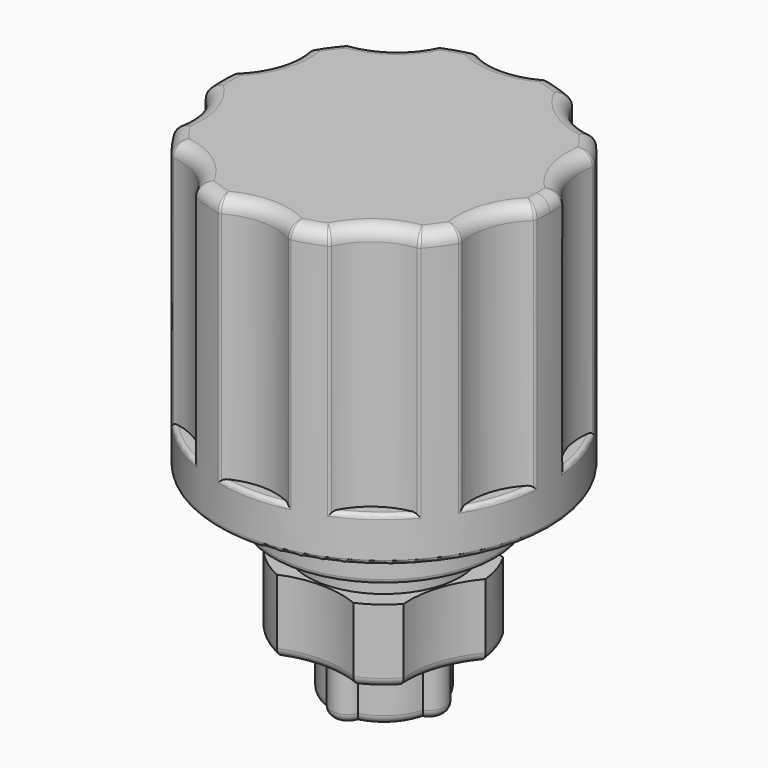
from build123d import *

# Parameters (mm, degrees)
F0_R         = 9.398
F1_DEPTH     = 16.51
F2_R         = 3.81
F3_DEPTH     = 13.97
F4_T2_ANGLE  = 17.4807543579
F4_T4_ANGLE  = 17.4807543579
F4_T6_ANGLE  = 119.7648433204
F4_T8_ANGLE  = 34.9616276293
F4_T10_ANGLE = 119.7648433204
F4_T12_ANGLE = 34.9616276293
F4_T14_ANGLE = 119.7648433204
F4_T16_ANGLE = 34.9616276293
F4_T18_ANGLE = 119.7648433204
F4_T20_ANGLE = 34.9616276293
F4_T22_ANGLE = 119.7648433204
F4_T24_ANGLE = 34.9616276293
F4_T26_ANGLE = 119.7648433204
F4_T28_ANGLE = 34.9616276293
F4_T30_ANGLE = 119.7648433204
F4_T32_ANGLE = 34.9616276293
F4_T34_ANGLE = 119.7648433204
F4_T36_ANGLE = 34.9616276293
F4_T38_ANGLE = 119.7648433204
F4_T40_ANGLE = 34.9616276293
F4_T42_ANGLE = 119.7648433204
F5_R         = 5.334
F6_DEPTH     = 8.255
F7_R         = 5.715
F8_DEPTH     = 7.62
F9_R         = 6.223
F9_R_2       = 4.3172960793
F10_DEPTH    = 4.064
F11_R        = 6.35
F12_DEPTH    = 2.54
F13_R        = 0.508
F14_R        = 0.254
F15_R        = 1.524
F16_DEPTH    = 10.414
F17_R        = 1.524
F18_DEPTH    = 3.048
F19_R        = 0.508


# Not quite as in the source:
# - a fillet or chamfer that OpenCascade refuses, or shapes differently, is made with other operations: its cross-section is extruded or revolved along the edge and cut away or added


with BuildPart() as f1:
    # F0 (on Top) → F1 (new body)
    with BuildSketch(Plane.XY):
        Circle(F0_R)
    extrude(amount=F1_DEPTH)

    # F2 (on face) → F3 (cut)
    with BuildSketch(Plane.XY.offset(16.51)):
        with Locations((-7.31557525, 10.069025512)):
            Circle(F2_R)
        with Locations((-11.8368494018, 3.846025512)):
            Circle(F2_R)
        with Locations((-11.8368494018, -3.846025512)):
            Circle(F2_R)
        with Locations((-7.31557525, -10.069025512)):
            Circle(F2_R)
        with Locations((0, -12.446)):
            Circle(F2_R)
        with Locations((7.31557525, -10.069025512)):
            Circle(F2_R)
        with Locations((11.8368494018, -3.846025512)):
            Circle(F2_R)
        with Locations((11.8368494018, 3.846025512)):
            Circle(F2_R)
        with Locations((7.31557525, 10.069025512)):
            Circle(F2_R)
        with Locations((0, 12.446)):
            Circle(F2_R)
    extrude(amount=-F3_DEPTH, mode=Mode.SUBTRACT)

    # F4: fillet of radius 0.762 on 21 edges, made by hand

    # F4_s1 → F4_t2 (revolve, cut)
    with BuildSketch(Plane(origin=(0, 0, 0), x_dir=(0, 0, 1), z_dir=(-0.3003854292, -0.953817904, 0))):
        with BuildLine():
            ThreePointArc((15.748, -9.398), (16.2868153673, -9.1748153673), (16.51, -8.636))
            Line((16.51, -8.636), (16.51, -9.398))
            Line((16.51, -9.398), (15.748, -9.398))
        make_face()
    revolve(axis=Axis((0, 0, 16.51), (0, 0, 1)), revolution_arc=F4_T2_ANGLE, mode=Mode.SUBTRACT)

    # F4_s3 → F4_t4 (revolve, cut)
    with BuildSketch(Plane.XZ):
        with BuildLine():
            ThreePointArc((9.398, 15.748), (9.1748153673, 16.2868153673), (8.636, 16.51))
            Line((8.636, 16.51), (9.398, 16.51))
            Line((9.398, 16.51), (9.398, 15.748))
        make_face()
    revolve(axis=Axis((0, 0, 16.51), (0, 0, 1)), revolution_arc=F4_T4_ANGLE, mode=Mode.SUBTRACT)

    # F4_s5 → F4_t6 (revolve, cut)
    with BuildSketch(Plane(origin=(7.187265654, 8.0152842237, 0), x_dir=(0, 0, 1), z_dir=(0.6676041693, 0.7445164022, 0))):
        with BuildLine():
            ThreePointArc((15.748, 2.4351058624), (16.2868153673, 2.2119212297), (16.51, 1.6731058624))
            Line((16.51, 1.6731058624), (16.51, 2.4351058624))
            Line((16.51, 2.4351058624), (15.748, 2.4351058624))
        make_face()
    revolve(axis=Axis((11.8368494018, 3.846025512, 16.51), (0, 0, 1)), revolution_arc=F4_T6_ANGLE, mode=Mode.SUBTRACT)

    # F4_s7 → F4_t8 (revolve, cut)
    with BuildSketch(Plane(origin=(0, 0, 0), x_dir=(0, 0, 1), z_dir=(0.3176221963, -0.9482173487, 0))):
        with BuildLine():
            ThreePointArc((15.748, -9.398), (16.2868153673, -9.1748153673), (16.51, -8.636))
            Line((16.51, -8.636), (16.51, -9.398))
            Line((16.51, -9.398), (15.748, -9.398))
        make_face()
    revolve(axis=Axis((0, 0, 16.51), (0, 0, 1)), revolution_arc=F4_T8_ANGLE, mode=Mode.SUBTRACT)

    # F4_s9 → F4_t10 (revolve, cut)
    with BuildSketch(Plane(origin=(1.1033541976, 10.7090699074, 0), x_dir=(0, 0, 1), z_dir=(0.1024873572, 0.994734307, 0))):
        with BuildLine():
            ThreePointArc((15.748, 2.4351058624), (16.2868153673, 2.2119212297), (16.51, 1.6731058624))
            Line((16.51, 1.6731058624), (16.51, 2.4351058624))
            Line((16.51, 2.4351058624), (15.748, 2.4351058624))
        make_face()
    revolve(axis=Axis((7.31557525, 10.069025512, 16.51), (0, 0, 1)), revolution_arc=F4_T10_ANGLE, mode=Mode.SUBTRACT)

    # F4_s11 → F4_t12 (revolve, cut)
    with BuildSketch(Plane(origin=(0, 0, 0), x_dir=(0, 0, 1), z_dir=(0.8143099281, -0.5804303067, 0))):
        with BuildLine():
            ThreePointArc((15.748, -9.398), (16.2868153673, -9.1748153673), (16.51, -8.636))
            Line((16.51, -8.636), (16.51, -9.398))
            Line((16.51, -9.398), (15.748, -9.398))
        make_face()
    revolve(axis=Axis((0, 0, 16.51), (0, 0, 1)), revolution_arc=F4_T12_ANGLE, mode=Mode.SUBTRACT)

    # F4_s13 → F4_t14 (revolve, cut)
    with BuildSketch(Plane(origin=(-5.4020010607, 9.3123548744, 0), x_dir=(0, 0, 1), z_dir=(-0.5017761419, 0.8649975164, 0))):
        with BuildLine():
            ThreePointArc((15.748, 2.4351058624), (16.2868153673, 2.2119212297), (16.51, 1.6731058624))
            Line((16.51, 1.6731058624), (16.51, 2.4351058624))
            Line((16.51, 2.4351058624), (15.748, 2.4351058624))
        make_face()
    revolve(axis=Axis((0, 12.446, 16.51), (0, 0, 1)), revolution_arc=F4_T14_ANGLE, mode=Mode.SUBTRACT)

    # F4_s15 → F4_t16 (revolve, cut)
    with BuildSketch(Plane(origin=(0, 0, 0), x_dir=(0, 0, 1), z_dir=(0.9999589448, 0.0090613844, 0))):
        with BuildLine():
            ThreePointArc((15.748, -9.398), (16.2868153673, -9.1748153673), (16.51, -8.636))
            Line((16.51, -8.636), (16.51, -9.398))
            Line((16.51, -9.398), (15.748, -9.398))
        make_face()
    revolve(axis=Axis((0, 0, 16.51), (0, 0, 1)), revolution_arc=F4_T16_ANGLE, mode=Mode.SUBTRACT)

    # F4_s17 → F4_t18 (revolve, cut)
    with BuildSketch(Plane(origin=(-9.843975521, 4.3586367947, 0), x_dir=(0, 0, 1), z_dir=(-0.9143782096, 0.4048610747, 0))):
        with BuildLine():
            ThreePointArc((15.748, 2.4351058624), (16.2868153673, 2.2119212297), (16.51, 1.6731058624))
            Line((16.51, 1.6731058624), (16.51, 2.4351058624))
            Line((16.51, 2.4351058624), (15.748, 2.4351058624))
        make_face()
    revolve(axis=Axis((-7.31557525, 10.069025512, 16.51), (0, 0, 1)), revolution_arc=F4_T18_ANGLE, mode=Mode.SUBTRACT)

    # F4_s19 → F4_t20 (revolve, cut)
    with BuildSketch(Plane(origin=(0, 0, 0), x_dir=(0, 0, 1), z_dir=(0.8036576319, 0.5950919346, 0))):
        with BuildLine():
            ThreePointArc((15.748, -9.398), (16.2868153673, -9.1748153673), (16.51, -8.636))
            Line((16.51, -8.636), (16.51, -9.398))
            Line((16.51, -9.398), (15.748, -9.398))
        make_face()
    revolve(axis=Axis((0, 0, 16.51), (0, 0, 1)), revolution_arc=F4_T20_ANGLE, mode=Mode.SUBTRACT)

    # F4_s21 → F4_t22 (revolve, cut)
    with BuildSketch(Plane(origin=(-7.187265654, 8.0152842237, 0), x_dir=(0, 0, 1), z_dir=(-0.6676041693, 0.7445164022, 0))):
        with BuildLine():
            ThreePointArc((15.748, -2.4351058624), (16.2868153673, -2.2119212297), (16.51, -1.6731058624))
            Line((16.51, -1.6731058624), (16.51, -2.4351058624))
            Line((16.51, -2.4351058624), (15.748, -2.4351058624))
        make_face()
    revolve(axis=Axis((-11.8368494018, 3.846025512, 16.51), (0, 0, -1)), revolution_arc=F4_T22_ANGLE, mode=Mode.SUBTRACT)

    # F4_s23 → F4_t24 (revolve, cut)
    with BuildSketch(Plane(origin=(0, 0, 0), x_dir=(0, 0, 1), z_dir=(0.300386419, 0.9538175923, 0))):
        with BuildLine():
            ThreePointArc((15.748, -9.398), (16.2868153673, -9.1748153673), (16.51, -8.636))
            Line((16.51, -8.636), (16.51, -9.398))
            Line((16.51, -9.398), (15.748, -9.398))
        make_face()
    revolve(axis=Axis((0, 0, 16.51), (0, 0, 1)), revolution_arc=F4_T24_ANGLE, mode=Mode.SUBTRACT)

    # F4_s25 → F4_t26 (revolve, cut)
    with BuildSketch(Plane(origin=(-10.5258859168, 2.259932396, 0), x_dir=(0, 0, 1), z_dir=(-0.9777188798, 0.2099185368, 0))):
        with BuildLine():
            ThreePointArc((15.748, -2.4351058624), (16.2868153673, -2.2119212297), (16.51, -1.6731058624))
            Line((16.51, -1.6731058624), (16.51, -2.4351058624))
            Line((16.51, -2.4351058624), (15.748, -2.4351058624))
        make_face()
    revolve(axis=Axis((-11.8368494018, -3.846025512, 16.51), (0, 0, -1)), revolution_arc=F4_T26_ANGLE, mode=Mode.SUBTRACT)

    # F4_s27 → F4_t28 (revolve, cut)
    with BuildSketch(Plane(origin=(0, 0, 0), x_dir=(0, 0, 1), z_dir=(-0.3176221963, 0.9482173487, 0))):
        with BuildLine():
            ThreePointArc((15.748, -9.398), (16.2868153673, -9.1748153673), (16.51, -8.636))
            Line((16.51, -8.636), (16.51, -9.398))
            Line((16.51, -9.398), (15.748, -9.398))
        make_face()
    revolve(axis=Axis((0, 0, 16.51), (0, 0, 1)), revolution_arc=F4_T28_ANGLE, mode=Mode.SUBTRACT)

    # F4_s29 → F4_t30 (revolve, cut)
    with BuildSketch(Plane(origin=(-1.1033541976, -10.7090699074, 0), x_dir=(0, 0, 1), z_dir=(-0.1024873572, -0.994734307, 0))):
        with BuildLine():
            ThreePointArc((15.748, 2.4351058624), (16.2868153673, 2.2119212297), (16.51, 1.6731058624))
            Line((16.51, 1.6731058624), (16.51, 2.4351058624))
            Line((16.51, 2.4351058624), (15.748, 2.4351058624))
        make_face()
    revolve(axis=Axis((-7.31557525, -10.069025512, 16.51), (0, 0, 1)), revolution_arc=F4_T30_ANGLE, mode=Mode.SUBTRACT)

    # F4_s31 → F4_t32 (revolve, cut)
    with BuildSketch(Plane(origin=(0, 0, 0), x_dir=(0, 0, 1), z_dir=(-0.8143099281, 0.5804303067, 0))):
        with BuildLine():
            ThreePointArc((15.748, -9.398), (16.2868153673, -9.1748153673), (16.51, -8.636))
            Line((16.51, -8.636), (16.51, -9.398))
            Line((16.51, -9.398), (15.748, -9.398))
        make_face()
    revolve(axis=Axis((0, 0, 16.51), (0, 0, 1)), revolution_arc=F4_T32_ANGLE, mode=Mode.SUBTRACT)

    # F4_s33 → F4_t34 (revolve, cut)
    with BuildSketch(Plane(origin=(5.4020010607, -9.3123548744, 0), x_dir=(0, 0, 1), z_dir=(0.5017761419, -0.8649975164, 0))):
        with BuildLine():
            ThreePointArc((15.748, 2.4351058624), (16.2868153673, 2.2119212297), (16.51, 1.6731058624))
            Line((16.51, 1.6731058624), (16.51, 2.4351058624))
            Line((16.51, 2.4351058624), (15.748, 2.4351058624))
        make_face()
    revolve(axis=Axis((0, -12.446, 16.51), (0, 0, 1)), revolution_arc=F4_T34_ANGLE, mode=Mode.SUBTRACT)

    # F4_s35 → F4_t36 (revolve, cut)
    with BuildSketch(Plane(origin=(0, 0, 0), x_dir=(0, 0, 1), z_dir=(-0.9999589448, -0.0090613844, 0))):
        with BuildLine():
            ThreePointArc((15.748, -9.398), (16.2868153673, -9.1748153673), (16.51, -8.636))
            Line((16.51, -8.636), (16.51, -9.398))
            Line((16.51, -9.398), (15.748, -9.398))
        make_face()
    revolve(axis=Axis((0, 0, 16.51), (0, 0, 1)), revolution_arc=F4_T36_ANGLE, mode=Mode.SUBTRACT)

    # F4_s37 → F4_t38 (revolve, cut)
    with BuildSketch(Plane(origin=(9.843975521, -4.3586367947, 0), x_dir=(0, 0, 1), z_dir=(0.9143782096, -0.4048610747, 0))):
        with BuildLine():
            ThreePointArc((15.748, 2.4351058624), (16.2868153673, 2.2119212297), (16.51, 1.6731058624))
            Line((16.51, 1.6731058624), (16.51, 2.4351058624))
            Line((16.51, 2.4351058624), (15.748, 2.4351058624))
        make_face()
    revolve(axis=Axis((7.31557525, -10.069025512, 16.51), (0, 0, 1)), revolution_arc=F4_T38_ANGLE, mode=Mode.SUBTRACT)

    # F4_s39 → F4_t40 (revolve, cut)
    with BuildSketch(Plane(origin=(0, 0, 0), x_dir=(0, 0, 1), z_dir=(-0.8036576319, -0.5950919346, 0))):
        with BuildLine():
            ThreePointArc((15.748, -9.398), (16.2868153673, -9.1748153673), (16.51, -8.636))
            Line((16.51, -8.636), (16.51, -9.398))
            Line((16.51, -9.398), (15.748, -9.398))
        make_face()
    revolve(axis=Axis((0, 0, 16.51), (0, 0, 1)), revolution_arc=F4_T40_ANGLE, mode=Mode.SUBTRACT)

    # F4_s41 → F4_t42 (revolve, cut)
    with BuildSketch(Plane(origin=(10.5258859168, 2.259932396, 0), x_dir=(0, 0, 1), z_dir=(0.9777188798, 0.2099185368, 0))):
        with BuildLine():
            ThreePointArc((15.748, 2.4351058624), (16.2868153673, 2.2119212297), (16.51, 1.6731058624))
            Line((16.51, 1.6731058624), (16.51, 2.4351058624))
            Line((16.51, 2.4351058624), (15.748, 2.4351058624))
        make_face()
    revolve(axis=Axis((11.8368494018, -3.846025512, 16.51), (0, 0, 1)), revolution_arc=F4_T42_ANGLE, mode=Mode.SUBTRACT)

    # F5 (on face) → F6 (join)
    with BuildSketch(Plane(origin=(0, 0, 0), x_dir=(1, 0, 0), z_dir=(0, 0, -1))):
        Circle(F5_R)
    extrude(amount=F6_DEPTH)

    # F7 (on face) → F8 (cut)
    with BuildSketch(Plane(origin=(0, 0, -8.255), x_dir=(1, 0, 0), z_dir=(0, 0, -1))):
        with Locations((0, 10.16)):
            Circle(F7_R)
        with Locations((-9.6627342056, 3.1396126628)):
            Circle(F7_R)
        with Locations((-5.9718981633, -8.2196126628)):
            Circle(F7_R)
        with Locations((5.9718981633, -8.2196126628)):
            Circle(F7_R)
        with Locations((9.6627342056, 3.1396126628)):
            Circle(F7_R)
    extrude(amount=-F8_DEPTH, mode=Mode.SUBTRACT)

    # F9 (on face) → F10 (cut)
    with BuildSketch(Plane(origin=(0, 0, 0), x_dir=(1, 0, 0), z_dir=(0, 0, -1))):
        Circle(F9_R)
        Circle(F9_R_2, mode=Mode.SUBTRACT)
    extrude(amount=F10_DEPTH, mode=Mode.SUBTRACT)

    # F11 (on face) → F12 (join)
    with BuildSketch(Plane(origin=(0, 0, 0), x_dir=(1, 0, 0), z_dir=(0, 0, -1))):
        Circle(F11_R)
    extrude(amount=F12_DEPTH)

    # F13
    f13_edges = [f1.edges().sort_by_distance(p)[0] for p in [
        (4.227446, -1.373581, -8.255),
        (3.135247, -4.315297, -8.255),
        (0, -4.445, -8.255),
        (-3.135247, -4.315297, -8.255),
        (-4.227446, -1.373581, -8.255),
        (-5.072935, 1.648297, -8.255),
        (-2.612705, 3.596081, -8.255),
        (0, 5.334, -8.255),
        (2.612705, 3.596081, -8.255),
        (5.072935, 1.648297, -8.255),
    ]]
    fillet(f13_edges, radius=F13_R)

    # F14
    f14_edges = [f1.edges().sort_by_distance(p)[0] for p in [
        (-6.35, 0, -2.54),
        (-9.398, 0, 0),
        (-5.524006, -7.603142, 2.54),
        (0, -9.398, 2.54),
        (-3.80253, -8.594368, 9.144),
        (-6.998684, -6.272227, 9.144),
        (1.975332, -9.188061, 9.144),
        (-1.975332, -9.188061, 9.144),
        (6.998684, -6.272227, 9.144),
        (3.80253, -8.594368, 9.144),
        (5.524006, -7.603142, 2.54),
        (9.348777, -0.960615, 9.144),
        (8.127954, -4.717919, 9.144),
        (8.938029, -2.904142, 2.54),
        (8.938029, 2.904142, 2.54),
        (8.127954, 4.717919, 9.144),
        (9.348777, 0.960615, 9.144),
        (3.80253, 8.594368, 9.144),
        (6.998684, 6.272227, 9.144),
        (5.524006, 7.603142, 2.54),
        (-1.975332, 9.188061, 9.144),
        (1.975332, 9.188061, 9.144),
        (0, 9.398, 2.54),
        (-5.524006, 7.603142, 2.54),
        (-6.998684, 6.272227, 9.144),
        (-3.80253, 8.594368, 9.144),
        (-9.348777, 0.960615, 9.144),
        (-8.127954, 4.717919, 9.144),
        (-8.938029, 2.904142, 2.54),
        (-8.127954, -4.717919, 9.144),
        (-9.348777, -0.960615, 9.144),
        (-8.938029, -2.904142, 2.54),
        (9.133021, -0.850289, 16.289105),
        (9.133021, 0.850289, 16.289105),
        (6.888982, -6.056154, 16.289104),
        (7.888575, -4.68036, 16.289087),
        (2.013586, -8.948773, 16.289104),
        (3.630931, -8.423265, 16.289105),
        (-3.630932, -8.423266, 16.289104),
        (-2.013583, -8.948791, 16.289087),
        (-6.888982, -6.056153, 16.289105),
        (-7.888556, -4.680357, 16.289105),
        (-9.133021, -0.850289, 16.289105),
        (-9.13302, 0.850289, 16.289105),
        (-6.888981, 6.056153, 16.289105),
        (-7.888556, 4.680357, 16.289105),
        (-2.013586, 8.948772, 16.289105),
        (-3.630931, 8.423265, 16.289105),
        (3.630932, 8.423266, 16.289104),
        (2.013586, 8.948772, 16.289105),
        (7.888556, 4.680357, 16.289105),
        (6.888982, 6.056153, 16.289105),
    ]]
    fillet(f14_edges, radius=F14_R)

    # F15 (on face) → F16 (cut)
    with BuildSketch(Plane(origin=(0, 0, -8.255), x_dir=(1, 0, 0), z_dir=(0, 0, -1))):
        Circle(F15_R)
    extrude(amount=-F16_DEPTH, mode=Mode.SUBTRACT)

    # F17 (on face) → F18 (join)
    with BuildSketch(Plane(origin=(0, 0, -8.255), x_dir=(1, 0, 0), z_dir=(0, 0, -1))):
        with BuildLine():
            ThreePointArc((-0.8733266614, -2.92020625), (0, -3.4925), (0.8733266614, -2.92020625))
            ThreePointArc((0.8733266614, -2.92020625), (2.1552614691, -2.1552614691), (2.92020625, -0.8733266614))
            ThreePointArc((2.92020625, -0.8733266614), (3.048, 0), (2.92020625, 0.8733266614))
            ThreePointArc((2.92020625, 0.8733266614), (2.1552614691, 2.1552614691), (0.8733266614, 2.92020625))
            ThreePointArc((0.8733266614, 2.92020625), (0, 3.048), (-0.8733266614, 2.92020625))
            ThreePointArc((-0.8733266614, 2.92020625), (-2.1552614691, 2.1552614691), (-2.92020625, 0.8733266614))
            ThreePointArc((-2.92020625, 0.8733266614), (-3.048, 0), (-2.92020625, -0.8733266614))
            ThreePointArc((-2.92020625, -0.8733266614), (-2.1552614691, -2.1552614691), (-0.8733266614, -2.92020625))
        make_face()
        Circle(F17_R, mode=Mode.SUBTRACT)
        with BuildLine():
            ThreePointArc((2.92020625, 0.8733266614), (3.048, 0), (2.92020625, -0.8733266614))
            ThreePointArc((2.92020625, -0.8733266614), (3.4925, 0), (2.92020625, 0.8733266614))
        make_face()
        with BuildLine():
            ThreePointArc((-2.92020625, 0.8733266614), (-3.4925, 0), (-2.92020625, -0.8733266614))
            ThreePointArc((-2.92020625, -0.8733266614), (-3.048, 0), (-2.92020625, 0.8733266614))
        make_face()
        with BuildLine():
            ThreePointArc((-0.8733266614, 2.92020625), (0, 3.048), (0.8733266614, 2.92020625))
            ThreePointArc((0.8733266614, 2.92020625), (0, 3.4925), (-0.8733266614, 2.92020625))
        make_face()
    extrude(amount=F18_DEPTH)

    # F19
    f19_edges = [f1.edges().sort_by_distance(p)[0] for p in [
        (0, 3.4925, -11.303),
        (2.155261, 2.155261, -11.303),
        (3.4925, 0, -11.303),
        (2.155261, -2.155261, -11.303),
        (0, -3.4925, -11.303),
        (-2.155261, -2.155261, -11.303),
        (-3.4925, 0, -11.303),
        (-2.155261, 2.155261, -11.303),
        (-1.524, 0, -11.303),
    ]]
    fillet(f19_edges, radius=F19_R)


solid = f1.part
